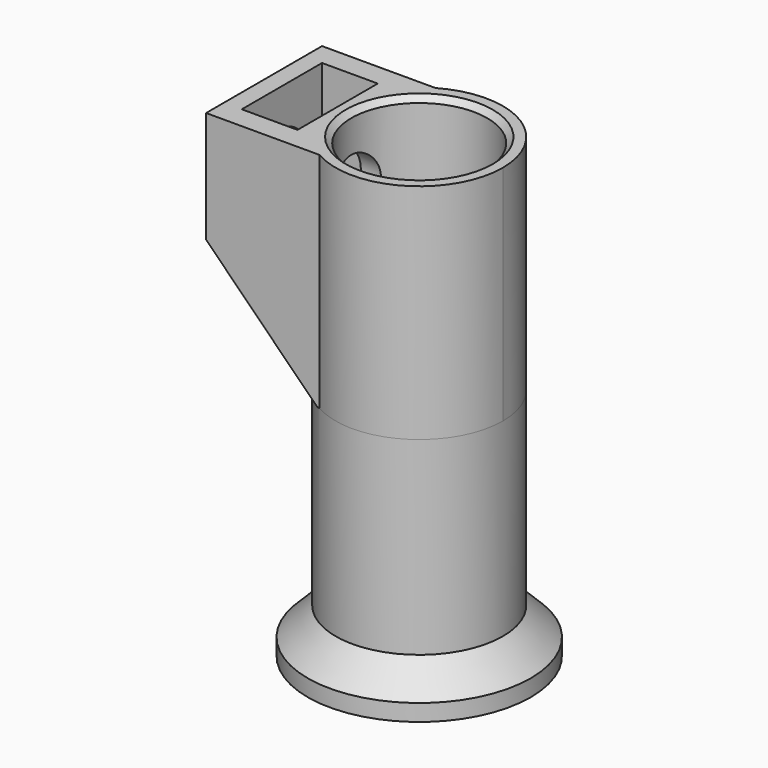
from build123d import *

# Parameters (mm, degrees)
F0_R         = 12.7
F0_R_2       = 3.429
F1_DEPTH     = 5.08
F2_SIZE      = 3.175
F3_DEPTH     = 1.27
F4_R         = 9.525
F4_R_2       = 7.747
F5_DEPTH     = 20.32
F6_R         = 7.747
F7_DEPTH     = 25.4
F8_T4_DEPTH  = 81.8307478943
F8_S5_R      = 9.525
F8_T6_DEPTH  = 43
F9_W         = 6.35
F9_H         = 11.43
F10_DEPTH    = 14.224
F11_T1_DEPTH = 6.35
F12_R        = 3.302
F13_DEPTH    = 12.7
F14_SIZE     = 0.635


# Not quite as in the source:
# - a fillet or chamfer that OpenCascade refuses, or shapes differently, is made with other operations: its cross-section is extruded or revolved along the edge and cut away or added


with BuildPart() as f1:
    # F0 (on Top) → F1 (new body)
    with BuildSketch(Plane.XY):
        Circle(F0_R)
        Circle(F0_R_2, mode=Mode.SUBTRACT)
    extrude(amount=F1_DEPTH)

    # F2
    f2_edges = [f1.edges().sort_by_distance(p)[0] for p in [
        (-12.7, 0, 5.08),
    ]]
    chamfer(f2_edges, length=F2_SIZE)

    # F3 (add): a face of the model
    f3_faces = [f1.faces().sort_by_distance(p)[0] for p in [
        (-9.2555923164, 0, 5.08),
    ]]
    extrude(f3_faces, amount=F3_DEPTH)

    # F4 (on face) → F5 (join)
    with BuildSketch(Plane.XY.offset(6.35)):
        Circle(F4_R)
        Circle(F4_R_2, mode=Mode.SUBTRACT)
    extrude(amount=F5_DEPTH)

    # F6 (on face) → F7 (join)
    with BuildSketch(Plane.XY.offset(26.67)):
        with BuildLine():
            ThreePointArc((9.525, 0), (4.7677946163, 8.2458328565), (-4.7519048812, 8.255))
            ThreePointArc((-4.7519048812, 8.255), (-9.525, 0), (-4.7519048812, -8.255))
            ThreePointArc((-4.7519048812, -8.255), (4.7677946163, -8.2458328565), (9.525, 0))
        make_face()
        Circle(F6_R, mode=Mode.SUBTRACT)
        with BuildLine():
            ThreePointArc((-4.7519048812, -8.255), (-9.525, 0), (-4.7519048812, 8.255))
            Line((-4.7519048812, 8.255), (-17.6784, 8.255))
            Line((-17.6784, 8.255), (-17.6784, -8.255))
            Line((-17.6784, -8.255), (-4.7519048812, -8.255))
        make_face()
    extrude(amount=F7_DEPTH)

    # F8: chamfer of 12.7 on 1 edges, made by hand


with BuildPart() as f8_tool2:
    # F8_s3 → F8_t4 (new body)
    with BuildSketch(Plane.XZ.offset(-40.9153739472)):
        Polygon((-4.9784, 26.67), (-17.6784, 39.37), (-17.6784, 26.67), align=None)
    extrude(amount=F8_T4_DEPTH)

    # F8_s5 → F8_t6 (cut, symmetric)
    with BuildSketch(Plane.XY.offset(33)):
        Circle(F8_S5_R)
    extrude(amount=F8_T6_DEPTH, both=True, mode=Mode.SUBTRACT)


with BuildPart() as f1_1:
    add(f1.part)

    # F8_t1: cut F8_tool2
    add(f8_tool2.part, mode=Mode.SUBTRACT)

    # F9 (on face) → F10 (cut)
    with BuildSketch(Plane.XY.offset(52.07)):
        with Locations((-12.4714, 0)):
            Rectangle(F9_W, F9_H)
    extrude(amount=-F10_DEPTH, mode=Mode.SUBTRACT)

    # F11: chamfer of 3.302 x 5.7192317666 on 2 edges, made by hand

    # F11_s2 → F11_t1 (join)
    with BuildSketch(Plane.YZ.offset(-15.6464)):
        Polygon((5.715, 41.148), (-0.0042317666, 37.846), (5.715, 37.846), align=None)
        Polygon((-5.715, 41.148), (0.0042317666, 37.846), (-5.715, 37.846), align=None)
    extrude(amount=F11_T1_DEPTH)

    # F12 (on face) → F13 (cut, symmetric)
    with BuildSketch(Plane.YZ.offset(-15.6464)):
        with Locations((0, 44.4475567884)):
            Circle(F12_R)
    extrude(amount=F13_DEPTH, both=True, mode=Mode.SUBTRACT)

    # F14
    f14_edges = [f1_1.edges().sort_by_distance(p)[0] for p in [
        (-7.747, 0, 52.07),
    ]]
    chamfer(f14_edges, length=F14_SIZE)


solid = f1_1.part
